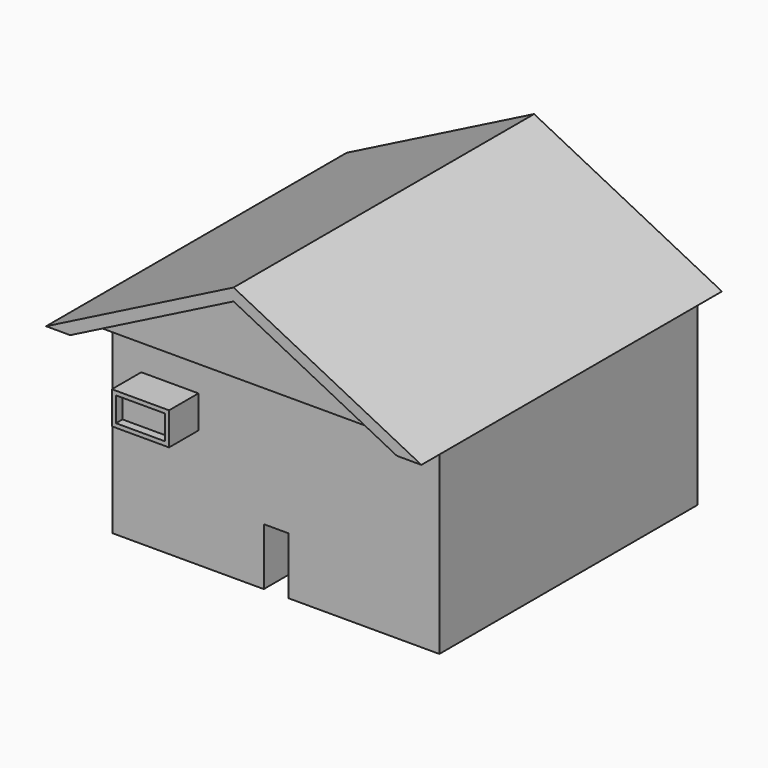
from build123d import *

# Parameters (mm, degrees)
F1_DEPTH = 14020.8
F2_DEPTH = 13106.4
F0_W     = 2133.6
F0_H     = 1219.2
F3_DEPTH = 12039.6
F0_W_2   = 1828.8
F0_H_2   = 914.4
F5_DEPTH = 13106.4
F6_DEPTH = 13411.2


# Not quite as in the source:
# - the program builds the solid bodies; features that only make, move or delete a surface that nothing else refers to are left out


with BuildPart() as f1:
    # F0 (on Front) → F1 (new body)
    with BuildSketch(Plane.XZ):
        Polygon((-6997.4747111522, 0), (-6096, 0), (0, 3091.7020361423), (0, 3548.9020361423), align=None)
        Polygon((0, 3548.9020361423), (0, 3091.7020361423), (6096, 0), (7010.4, 0), align=None)
    extrude(amount=F1_DEPTH)

    # F0 (on Front) → F2 (join)
    with BuildSketch(Plane.XZ):
        Polygon((0, 3091.7020361423), (-6096, 0), (0, 0), (6096, 0), align=None)
    extrude(amount=F2_DEPTH)

    # F0 (on Front) → F3 (join)
    with BuildSketch(Plane.XZ):
        Polygon((0, 0), (-6096, 0), (-6096, -7315.2), (-457.2, -7315.2), (-457.2, -5181.6), (457.2, -5181.6), (457.2, -7315.2), (6096, -7315.2), (6096, 0), align=None)
        with Locations((-3962.4, -2286)):
            Rectangle(F0_W, F0_H, mode=Mode.SUBTRACT)
    extrude(amount=F3_DEPTH)


with BuildPart() as f5:
    # F0 (on Front) → F5 (new body)
    with BuildSketch(Plane.XZ):
        with Locations((-3962.4, -2286)):
            Rectangle(F0_W_2, F0_H_2)
    extrude(amount=F5_DEPTH)


with BuildPart() as f6:
    # F0 (on Front) → F6 (new body)
    with BuildSketch(Plane.XZ):
        with Locations((-3962.4, -2286)):
            Rectangle(F0_W, F0_H)
        with Locations((-3962.4, -2286)):
            Rectangle(F0_W_2, F0_H_2, mode=Mode.SUBTRACT)
    extrude(amount=F6_DEPTH)


solid = Compound([f1.part, f5.part, f6.part])
